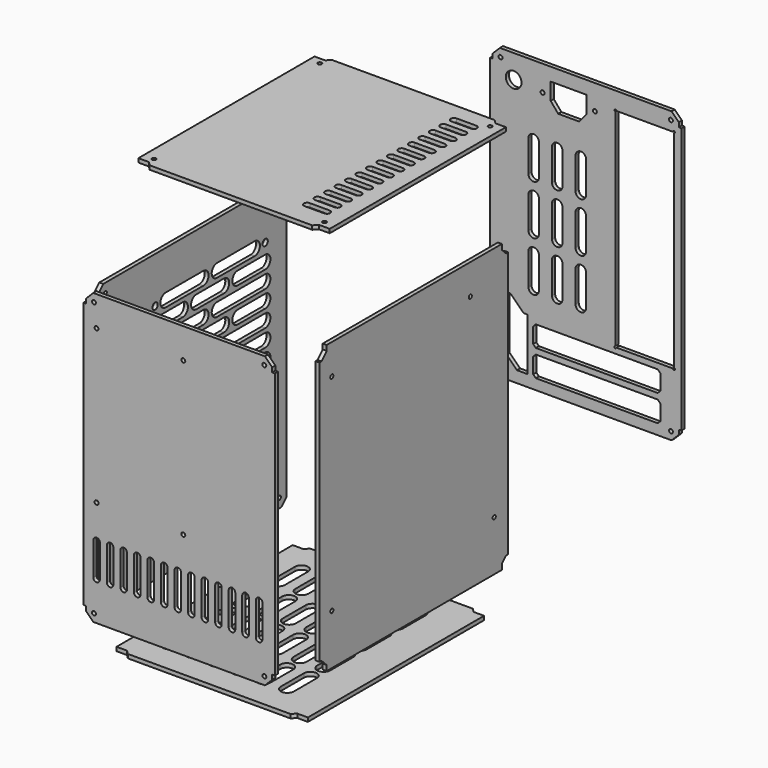
from build123d import *

# Parameters (mm, degrees)
F0_R      = 1.5
F1_DEPTH  = 3
F3_R      = 1.5
F4_DEPTH  = 3
F7_DEPTH  = 3
F9_R      = 1.5
F10_DEPTH = 25
F12_R     = 1.5
F13_DEPTH = 3
F15_R     = 2.5
F16_DEPTH = 25
F18_R     = 1.5
F19_DEPTH = 3
F23_DEPTH = 3
F27_DEPTH = 25
F28_R     = 1.5
F29_DEPTH = 3
F31_W     = 97
F31_H     = 15.9
F32_R     = 1.5
F32_R_2   = 6
F33_DEPTH = 25
F34_SIZE  = 2
F36_DEPTH = 25


# Not quite as in the source:
# - a feature names something its author has since deleted; it is built from what else it names


with BuildPart() as f1:
    # F0 (on Front) → F1 (new body)
    with BuildSketch(Plane.XZ):
        Polygon((-73.4445467208, 95.1760702261), (-75.4445467208, 95.1760702261), (-75.4445467208, -6.3239297739), (70.5554532792, -6.3239297739), (70.5554532792, 95.1760702261), (68.5554532792, 95.1760702261), (68.5554532792, 98.6760702261), (63.0554532792, 104.1760702261), (-67.9445467208, 104.1760702261), (-73.4445467208, 98.6760702261), align=None)
        with Locations((-67.4445467208, 98.1760702261)):
            Circle(F0_R, mode=Mode.SUBTRACT)
        with Locations((62.5554532792, 98.1760702261)):
            Circle(F0_R, mode=Mode.SUBTRACT)
    extrude(amount=F1_DEPTH)

    # F2: F1 across face


with BuildPart() as f1_1:
    add(f1.part)
    add(f1.part.mirror(Plane(origin=(-2.4445467208, -1.5, -6.3239297739), x_dir=(1, 0, 0), z_dir=(0, 0, -1))))

    # F3 (on face) → F4 (cut)
    with BuildSketch(Plane.XZ.offset(3)):
        with Locations((0.7554532792, 81.1760702261)):
            Circle(F3_R)
        with Locations((-65.4445467208, 81.1760702261)):
            Circle(F3_R)
        with Locations((-65.4445467208, -35.8239297739)):
            Circle(F3_R)
        with Locations((0.7554532792, -35.8239297739)):
            Circle(F3_R)
        with BuildLine():
            ThreePointArc((-67.9445467208, -86.8239297739), (-65.4445467208, -89.3239297739), (-62.9445467208, -86.8239297739))
            Line((-62.9445467208, -86.8239297739), (-62.9445467208, -61.8239297739))
            ThreePointArc((-62.9445467208, -61.8239297739), (-65.4445467208, -59.3239297739), (-67.9445467208, -61.8239297739))
            Line((-67.9445467208, -61.8239297739), (-67.9445467208, -86.8239297739))
        make_face()
        with BuildLine():
            ThreePointArc((-57.6115467208, -86.8239297739), (-55.1115467208, -89.3239297739), (-52.6115467208, -86.8239297739))
            Line((-52.6115467208, -86.8239297739), (-52.6115467208, -61.8239297739))
            ThreePointArc((-52.6115467208, -61.8239297739), (-55.1115467208, -59.3239297739), (-57.6115467208, -61.8239297739))
            Line((-57.6115467208, -61.8239297739), (-57.6115467208, -86.8239297739))
        make_face()
        with BuildLine():
            ThreePointArc((-47.2785467208, -86.8239297739), (-44.7785467208, -89.3239297739), (-42.2785467208, -86.8239297739))
            Line((-42.2785467208, -86.8239297739), (-42.2785467208, -61.8239297739))
            ThreePointArc((-42.2785467208, -61.8239297739), (-44.7785467208, -59.3239297739), (-47.2785467208, -61.8239297739))
            Line((-47.2785467208, -61.8239297739), (-47.2785467208, -86.8239297739))
        make_face()
        with BuildLine():
            ThreePointArc((-36.9455467208, -86.8239297739), (-34.4455467208, -89.3239297739), (-31.9455467208, -86.8239297739))
            Line((-31.9455467208, -86.8239297739), (-31.9455467208, -61.8239297739))
            ThreePointArc((-31.9455467208, -61.8239297739), (-34.4455467208, -59.3239297739), (-36.9455467208, -61.8239297739))
            Line((-36.9455467208, -61.8239297739), (-36.9455467208, -86.8239297739))
        make_face()
        with BuildLine():
            ThreePointArc((-26.6125467208, -86.8239297739), (-24.1125467208, -89.3239297739), (-21.6125467208, -86.8239297739))
            Line((-21.6125467208, -86.8239297739), (-21.6125467208, -61.8239297739))
            ThreePointArc((-21.6125467208, -61.8239297739), (-24.1125467208, -59.3239297739), (-26.6125467208, -61.8239297739))
            Line((-26.6125467208, -61.8239297739), (-26.6125467208, -86.8239297739))
        make_face()
        with BuildLine():
            ThreePointArc((-16.2795467208, -86.8239297739), (-13.7795467208, -89.3239297739), (-11.2795467208, -86.8239297739))
            Line((-11.2795467208, -86.8239297739), (-11.2795467208, -61.8239297739))
            ThreePointArc((-11.2795467208, -61.8239297739), (-13.7795467208, -59.3239297739), (-16.2795467208, -61.8239297739))
            Line((-16.2795467208, -61.8239297739), (-16.2795467208, -86.8239297739))
        make_face()
        with BuildLine():
            ThreePointArc((-5.9465467208, -86.8239297739), (-3.4465467208, -89.3239297739), (-0.9465467208, -86.8239297739))
            Line((-0.9465467208, -86.8239297739), (-0.9465467208, -61.8239297739))
            ThreePointArc((-0.9465467208, -61.8239297739), (-3.4465467208, -59.3239297739), (-5.9465467208, -61.8239297739))
            Line((-5.9465467208, -61.8239297739), (-5.9465467208, -86.8239297739))
        make_face()
        with BuildLine():
            ThreePointArc((4.3864532792, -86.8239297739), (6.8864532792, -89.3239297739), (9.3864532792, -86.8239297739))
            Line((9.3864532792, -86.8239297739), (9.3864532792, -61.8239297739))
            ThreePointArc((9.3864532792, -61.8239297739), (6.8864532792, -59.3239297739), (4.3864532792, -61.8239297739))
            Line((4.3864532792, -61.8239297739), (4.3864532792, -86.8239297739))
        make_face()
        with BuildLine():
            ThreePointArc((14.7194532792, -86.8239297739), (17.2194532792, -89.3239297739), (19.7194532792, -86.8239297739))
            Line((19.7194532792, -86.8239297739), (19.7194532792, -61.8239297739))
            ThreePointArc((19.7194532792, -61.8239297739), (17.2194532792, -59.3239297739), (14.7194532792, -61.8239297739))
            Line((14.7194532792, -61.8239297739), (14.7194532792, -86.8239297739))
        make_face()
        with BuildLine():
            ThreePointArc((25.0524532792, -86.8239297739), (27.5524532792, -89.3239297739), (30.0524532792, -86.8239297739))
            Line((30.0524532792, -86.8239297739), (30.0524532792, -61.8239297739))
            ThreePointArc((30.0524532792, -61.8239297739), (27.5524532792, -59.3239297739), (25.0524532792, -61.8239297739))
            Line((25.0524532792, -61.8239297739), (25.0524532792, -86.8239297739))
        make_face()
        with BuildLine():
            ThreePointArc((35.3854532792, -86.8239297739), (37.8854532792, -89.3239297739), (40.3854532792, -86.8239297739))
            Line((40.3854532792, -86.8239297739), (40.3854532792, -61.8239297739))
            ThreePointArc((40.3854532792, -61.8239297739), (37.8854532792, -59.3239297739), (35.3854532792, -61.8239297739))
            Line((35.3854532792, -61.8239297739), (35.3854532792, -86.8239297739))
        make_face()
        with BuildLine():
            ThreePointArc((45.7184532792, -86.8239297739), (48.2184532792, -89.3239297739), (50.7184532792, -86.8239297739))
            Line((50.7184532792, -86.8239297739), (50.7184532792, -61.8239297739))
            ThreePointArc((50.7184532792, -61.8239297739), (48.2184532792, -59.3239297739), (45.7184532792, -61.8239297739))
            Line((45.7184532792, -61.8239297739), (45.7184532792, -86.8239297739))
        make_face()
        with BuildLine():
            ThreePointArc((56.0514532792, -86.8239297739), (58.5514532792, -89.3239297739), (61.0514532792, -86.8239297739))
            Line((61.0514532792, -86.8239297739), (61.0514532792, -61.8239297739))
            ThreePointArc((61.0514532792, -61.8239297739), (58.5514532792, -59.3239297739), (56.0514532792, -61.8239297739))
            Line((56.0514532792, -61.8239297739), (56.0514532792, -86.8239297739))
        make_face()
    extrude(amount=-F4_DEPTH, mode=Mode.SUBTRACT)


with BuildPart() as f7:
    # F6 (on offset) → F7 (new body)
    with BuildSketch(Plane.YZ.offset(80)):
        Polygon((197.9221091728, 104.5042446256), (30.9221091728, 104.5042446256), (30.9221091728, 100.5042446256), (25.9221091728, 95.5042446256), (23.9221091728, 95.5042446256), (23.9221091728, -4.9957553744), (203.9221091728, -4.9957553744), (203.9221091728, 96.5042446256), (201.9221091728, 96.5042446256), (197.9221091728, 100.5042446256), align=None)
    extrude(amount=F7_DEPTH)

    # F8: F7 across face


with BuildPart() as f7_1:
    add(f7.part)
    add(f7.part.mirror(Plane(origin=(81.5, 113.9221091728, -4.9957553744), x_dir=(1, 0, 0), z_dir=(0, 0, -1))))

    # F9 (on face) → F10 (cut)
    with BuildSketch(Plane(origin=(80, 0, 0), x_dir=(0, -1, 0), z_dir=(-1, 0, 0))):
        with Locations((-190.7221091728, -76.0957553744)):
            Circle(F9_R)
        with Locations((-35.8221091728, -76.0957553744)):
            Circle(F9_R)
        with Locations((-167.9221091728, 81.3042446256)):
            Circle(F9_R)
        with Locations((-35.8221091728, 81.3042446256)):
            Circle(F9_R)
    extrude(amount=-F10_DEPTH, mode=Mode.SUBTRACT)


with BuildPart() as f13:
    # F12 (on offset) → F13 (new body)
    with BuildSketch(Plane.YZ.offset(-96)):
        Polygon((212.7864820957, 80.4807467597), (207.7864820957, 85.4807467597), (37.7864820957, 85.4807467597), (32.7864820957, 80.4807467597), (32.7864820957, -24.0192532403), (212.7864820957, -24.0192532403), align=None)
        with Locations((39.7864820957, 78.4807467597)):
            Circle(F12_R, mode=Mode.SUBTRACT)
        with Locations((205.7864820957, 78.4807467597)):
            Circle(F12_R, mode=Mode.SUBTRACT)
    extrude(amount=F13_DEPTH)

    # F14: F13 across face


with BuildPart() as f13_1:
    add(f13.part)
    add(f13.part.mirror(Plane(origin=(-94.5, 122.7864820957, -24.0192532403), x_dir=(1, 0, 0), z_dir=(0, 0, -1))))

    # F15 (on face) → F16 (cut)
    with BuildSketch(Plane(origin=(-96, 0, 0), x_dir=(0, -1, 0), z_dir=(-1, 0, 0))):
        with Locations((-192.2864820957, 50.4807467597)):
            Circle(F15_R)
        with Locations((-87.2864820957, 50.4807467597)):
            Circle(F15_R)
        with BuildLine():
            ThreePointArc((-182.2864820957, 55.4807467597), (-187.2864820957, 50.4807467597), (-182.2864820957, 45.4807467597))
            Line((-182.2864820957, 45.4807467597), (-146.2864820957, 45.4807467597))
            ThreePointArc((-146.2864820957, 45.4807467597), (-141.2864820957, 50.4807467597), (-146.2864820957, 55.4807467597))
            Line((-146.2864820957, 55.4807467597), (-182.2864820957, 55.4807467597))
        make_face()
        with BuildLine():
            ThreePointArc((-133.2864820957, 55.4807467597), (-138.2864820957, 50.4807467597), (-133.2864820957, 45.4807467597))
            Line((-133.2864820957, 45.4807467597), (-97.2864820957, 45.4807467597))
            ThreePointArc((-97.2864820957, 45.4807467597), (-92.2864820957, 50.4807467597), (-97.2864820957, 55.4807467597))
            Line((-97.2864820957, 55.4807467597), (-133.2864820957, 55.4807467597))
        make_face()
        with BuildLine():
            ThreePointArc((-192.2864820957, 42.3557467597), (-197.2864820957, 37.3557467597), (-192.2864820957, 32.3557467597))
            Line((-192.2864820957, 32.3557467597), (-165.9531487624, 32.3557467597))
            ThreePointArc((-165.9531487624, 32.3557467597), (-160.9531487624, 37.3557467597), (-165.9531487624, 42.3557467597))
            Line((-165.9531487624, 42.3557467597), (-192.2864820957, 42.3557467597))
        make_face()
        with BuildLine():
            ThreePointArc((-152.9531487624, 42.3557467597), (-157.9531487624, 37.3557467597), (-152.9531487624, 32.3557467597))
            Line((-152.9531487624, 32.3557467597), (-126.6198154291, 32.3557467597))
            ThreePointArc((-126.6198154291, 32.3557467597), (-121.6198154291, 37.3557467597), (-126.6198154291, 42.3557467597))
            Line((-126.6198154291, 42.3557467597), (-152.9531487624, 42.3557467597))
        make_face()
        with BuildLine():
            ThreePointArc((-113.6198154291, 42.3557467597), (-118.6198154291, 37.3557467597), (-113.6198154291, 32.3557467597))
            Line((-113.6198154291, 32.3557467597), (-87.2864820957, 32.3557467597))
            ThreePointArc((-87.2864820957, 32.3557467597), (-82.2864820957, 37.3557467597), (-87.2864820957, 42.3557467597))
            Line((-87.2864820957, 42.3557467597), (-113.6198154291, 42.3557467597))
        make_face()
        with BuildLine():
            ThreePointArc((-192.2864820957, 29.2307467597), (-197.2864820957, 24.2307467597), (-192.2864820957, 19.2307467597))
            Line((-192.2864820957, 19.2307467597), (-146.2864820957, 19.2307467597))
            ThreePointArc((-146.2864820957, 19.2307467597), (-141.2864820957, 24.2307467597), (-146.2864820957, 29.2307467597))
            Line((-146.2864820957, 29.2307467597), (-192.2864820957, 29.2307467597))
        make_face()
        with BuildLine():
            ThreePointArc((-133.2864820957, 29.2307467597), (-138.2864820957, 24.2307467597), (-133.2864820957, 19.2307467597))
            Line((-133.2864820957, 19.2307467597), (-87.2864820957, 19.2307467597))
            ThreePointArc((-87.2864820957, 19.2307467597), (-82.2864820957, 24.2307467597), (-87.2864820957, 29.2307467597))
            Line((-87.2864820957, 29.2307467597), (-133.2864820957, 29.2307467597))
        make_face()
        with BuildLine():
            ThreePointArc((-192.2864820957, 16.1057467597), (-197.2864820957, 11.1057467597), (-192.2864820957, 6.1057467597))
            Line((-192.2864820957, 6.1057467597), (-165.9531487624, 6.1057467597))
            ThreePointArc((-165.9531487624, 6.1057467597), (-160.9531487624, 11.1057467597), (-165.9531487624, 16.1057467597))
            Line((-165.9531487624, 16.1057467597), (-192.2864820957, 16.1057467597))
        make_face()
        with BuildLine():
            ThreePointArc((-152.9531487624, 16.1057467597), (-157.9531487624, 11.1057467597), (-152.9531487624, 6.1057467597))
            Line((-152.9531487624, 6.1057467597), (-126.6198154291, 6.1057467597))
            ThreePointArc((-126.6198154291, 6.1057467597), (-121.6198154291, 11.1057467597), (-126.6198154291, 16.1057467597))
            Line((-126.6198154291, 16.1057467597), (-152.9531487624, 16.1057467597))
        make_face()
        with BuildLine():
            ThreePointArc((-113.6198154291, 16.1057467597), (-118.6198154291, 11.1057467597), (-113.6198154291, 6.1057467597))
            Line((-113.6198154291, 6.1057467597), (-87.2864820957, 6.1057467597))
            ThreePointArc((-87.2864820957, 6.1057467597), (-82.2864820957, 11.1057467597), (-87.2864820957, 16.1057467597))
            Line((-87.2864820957, 16.1057467597), (-113.6198154291, 16.1057467597))
        make_face()
        with BuildLine():
            ThreePointArc((-192.2864820957, 2.9807467597), (-197.2864820957, -2.0192532403), (-192.2864820957, -7.0192532403))
            Line((-192.2864820957, -7.0192532403), (-146.2864820957, -7.0192532403))
            ThreePointArc((-146.2864820957, -7.0192532403), (-141.2864820957, -2.0192532403), (-146.2864820957, 2.9807467597))
            Line((-146.2864820957, 2.9807467597), (-192.2864820957, 2.9807467597))
        make_face()
        with BuildLine():
            ThreePointArc((-133.2864820957, 2.9807467597), (-138.2864820957, -2.0192532403), (-133.2864820957, -7.0192532403))
            Line((-133.2864820957, -7.0192532403), (-87.2864820957, -7.0192532403))
            ThreePointArc((-87.2864820957, -7.0192532403), (-82.2864820957, -2.0192532403), (-87.2864820957, 2.9807467597))
            Line((-87.2864820957, 2.9807467597), (-133.2864820957, 2.9807467597))
        make_face()
        with BuildLine():
            ThreePointArc((-192.2864820957, -10.1442532403), (-197.2864820957, -15.1442532403), (-192.2864820957, -20.1442532403))
            Line((-192.2864820957, -20.1442532403), (-165.9531487624, -20.1442532403))
            ThreePointArc((-165.9531487624, -20.1442532403), (-160.9531487624, -15.1442532403), (-165.9531487624, -10.1442532403))
            Line((-165.9531487624, -10.1442532403), (-192.2864820957, -10.1442532403))
        make_face()
        with BuildLine():
            ThreePointArc((-152.9531487624, -10.1442532403), (-157.9531487624, -15.1442532403), (-152.9531487624, -20.1442532403))
            Line((-152.9531487624, -20.1442532403), (-126.6198154291, -20.1442532403))
            ThreePointArc((-126.6198154291, -20.1442532403), (-121.6198154291, -15.1442532403), (-126.6198154291, -10.1442532403))
            Line((-126.6198154291, -10.1442532403), (-152.9531487624, -10.1442532403))
        make_face()
        with BuildLine():
            ThreePointArc((-113.6198154291, -10.1442532403), (-118.6198154291, -15.1442532403), (-113.6198154291, -20.1442532403))
            Line((-113.6198154291, -20.1442532403), (-87.2864820957, -20.1442532403))
            ThreePointArc((-87.2864820957, -20.1442532403), (-82.2864820957, -15.1442532403), (-87.2864820957, -10.1442532403))
            Line((-87.2864820957, -10.1442532403), (-113.6198154291, -10.1442532403))
        make_face()
        with BuildLine():
            ThreePointArc((-192.2864820957, -23.2692532403), (-197.2864820957, -28.2692532403), (-192.2864820957, -33.2692532403))
            Line((-192.2864820957, -33.2692532403), (-146.2864820957, -33.2692532403))
            ThreePointArc((-146.2864820957, -33.2692532403), (-141.2864820957, -28.2692532403), (-146.2864820957, -23.2692532403))
            Line((-146.2864820957, -23.2692532403), (-192.2864820957, -23.2692532403))
        make_face()
        with BuildLine():
            ThreePointArc((-133.2864820957, -23.2692532403), (-138.2864820957, -28.2692532403), (-133.2864820957, -33.2692532403))
            Line((-133.2864820957, -33.2692532403), (-87.2864820957, -33.2692532403))
            ThreePointArc((-87.2864820957, -33.2692532403), (-82.2864820957, -28.2692532403), (-87.2864820957, -23.2692532403))
            Line((-87.2864820957, -23.2692532403), (-133.2864820957, -23.2692532403))
        make_face()
        with BuildLine():
            ThreePointArc((-192.2864820957, -36.3942532403), (-197.2864820957, -41.3942532403), (-192.2864820957, -46.3942532403))
            Line((-192.2864820957, -46.3942532403), (-165.9531487624, -46.3942532403))
            ThreePointArc((-165.9531487624, -46.3942532403), (-160.9531487624, -41.3942532403), (-165.9531487624, -36.3942532403))
            Line((-165.9531487624, -36.3942532403), (-192.2864820957, -36.3942532403))
        make_face()
        with BuildLine():
            ThreePointArc((-152.9531487624, -36.3942532403), (-157.9531487624, -41.3942532403), (-152.9531487624, -46.3942532403))
            Line((-152.9531487624, -46.3942532403), (-126.6198154291, -46.3942532403))
            ThreePointArc((-126.6198154291, -46.3942532403), (-121.6198154291, -41.3942532403), (-126.6198154291, -36.3942532403))
            Line((-126.6198154291, -36.3942532403), (-152.9531487624, -36.3942532403))
        make_face()
        with BuildLine():
            ThreePointArc((-113.6198154291, -36.3942532403), (-118.6198154291, -41.3942532403), (-113.6198154291, -46.3942532403))
            Line((-113.6198154291, -46.3942532403), (-87.2864820957, -46.3942532403))
            ThreePointArc((-87.2864820957, -46.3942532403), (-82.2864820957, -41.3942532403), (-87.2864820957, -36.3942532403))
            Line((-87.2864820957, -36.3942532403), (-113.6198154291, -36.3942532403))
        make_face()
        with BuildLine():
            ThreePointArc((-182.2864820957, -49.5192532403), (-187.2864820957, -54.5192532403), (-182.2864820957, -59.5192532403))
            Line((-182.2864820957, -59.5192532403), (-146.2864820957, -59.5192532403))
            ThreePointArc((-146.2864820957, -59.5192532403), (-141.2864820957, -54.5192532403), (-146.2864820957, -49.5192532403))
            Line((-146.2864820957, -49.5192532403), (-182.2864820957, -49.5192532403))
        make_face()
        with BuildLine():
            ThreePointArc((-133.2864820957, -49.5192532403), (-138.2864820957, -54.5192532403), (-133.2864820957, -59.5192532403))
            Line((-133.2864820957, -59.5192532403), (-97.2864820957, -59.5192532403))
            ThreePointArc((-97.2864820957, -59.5192532403), (-92.2864820957, -54.5192532403), (-97.2864820957, -49.5192532403))
            Line((-97.2864820957, -49.5192532403), (-133.2864820957, -49.5192532403))
        make_face()
        with Locations((-192.2864820957, -54.5192532403)):
            Circle(F15_R)
        with Locations((-87.2864820957, -54.5192532403)):
            Circle(F15_R)
    extrude(amount=-F16_DEPTH, mode=Mode.SUBTRACT)


with BuildPart() as f19:
    # F18 (on offset) → F19 (new body)
    with BuildSketch(Plane.XY.offset(155)):
        Polygon((54.9777505851, 152.8661787467), (-91.0222494149, 152.8661787467), (-91.0222494149, 68.8661787467), (-83.0222494149, 68.8661787467), (-80.0222494149, 65.8661787467), (43.9777505851, 65.8661787467), (46.9777505851, 68.8661787467), (54.9777505851, 68.8661787467), align=None)
        with Locations((-83.0222494149, 73.8661787467)):
            Circle(F18_R, mode=Mode.SUBTRACT)
        with Locations((46.9777505851, 73.8661787467)):
            Circle(F18_R, mode=Mode.SUBTRACT)
    extrude(amount=F19_DEPTH)

    # F20: F19 across face


with BuildPart() as f19_1:
    add(f19.part)
    add(f19.part.mirror(Plane(origin=(-18.0222494149, 152.8661787467, 156.5), x_dir=(-1, 0, 0), z_dir=(0, 1, 0))))

    # F35 (on face) → F36 (cut)
    with BuildSketch(Plane.XY.offset(158)):
        with BuildLine():
            ThreePointArc((24.9777505851, 227.3661787467), (22.4777505851, 224.8661787467), (24.9777505851, 222.3661787467))
            Line((24.9777505851, 222.3661787467), (39.9777505851, 222.3661787467))
            ThreePointArc((39.9777505851, 222.3661787467), (42.4777505851, 224.8661787467), (39.9777505851, 227.3661787467))
            Line((39.9777505851, 227.3661787467), (24.9777505851, 227.3661787467))
        make_face()
        with BuildLine():
            ThreePointArc((24.9777505851, 217.3661787467), (22.4777505851, 214.8661787467), (24.9777505851, 212.3661787467))
            Line((24.9777505851, 212.3661787467), (39.9777505851, 212.3661787467))
            ThreePointArc((39.9777505851, 212.3661787467), (42.4777505851, 214.8661787467), (39.9777505851, 217.3661787467))
            Line((39.9777505851, 217.3661787467), (24.9777505851, 217.3661787467))
        make_face()
        with BuildLine():
            ThreePointArc((24.9777505851, 207.3661787467), (22.4777505851, 204.8661787467), (24.9777505851, 202.3661787467))
            Line((24.9777505851, 202.3661787467), (39.9777505851, 202.3661787467))
            ThreePointArc((39.9777505851, 202.3661787467), (42.4777505851, 204.8661787467), (39.9777505851, 207.3661787467))
            Line((39.9777505851, 207.3661787467), (24.9777505851, 207.3661787467))
        make_face()
        with BuildLine():
            ThreePointArc((24.9777505851, 197.3661787467), (22.4777505851, 194.8661787467), (24.9777505851, 192.3661787467))
            Line((24.9777505851, 192.3661787467), (39.9777505851, 192.3661787467))
            ThreePointArc((39.9777505851, 192.3661787467), (42.4777505851, 194.8661787467), (39.9777505851, 197.3661787467))
            Line((39.9777505851, 197.3661787467), (24.9777505851, 197.3661787467))
        make_face()
        with BuildLine():
            ThreePointArc((24.9777505851, 187.3661787467), (22.4777505851, 184.8661787467), (24.9777505851, 182.3661787467))
            Line((24.9777505851, 182.3661787467), (39.9777505851, 182.3661787467))
            ThreePointArc((39.9777505851, 182.3661787467), (42.4777505851, 184.8661787467), (39.9777505851, 187.3661787467))
            Line((39.9777505851, 187.3661787467), (24.9777505851, 187.3661787467))
        make_face()
        with BuildLine():
            ThreePointArc((24.9777505851, 177.3661787467), (22.4777505851, 174.8661787467), (24.9777505851, 172.3661787467))
            Line((24.9777505851, 172.3661787467), (39.9777505851, 172.3661787467))
            ThreePointArc((39.9777505851, 172.3661787467), (42.4777505851, 174.8661787467), (39.9777505851, 177.3661787467))
            Line((39.9777505851, 177.3661787467), (24.9777505851, 177.3661787467))
        make_face()
        with BuildLine():
            ThreePointArc((24.9777505851, 167.3661787467), (22.4777505851, 164.8661787467), (24.9777505851, 162.3661787467))
            Line((24.9777505851, 162.3661787467), (39.9777505851, 162.3661787467))
            ThreePointArc((39.9777505851, 162.3661787467), (42.4777505851, 164.8661787467), (39.9777505851, 167.3661787467))
            Line((39.9777505851, 167.3661787467), (24.9777505851, 167.3661787467))
        make_face()
        with BuildLine():
            ThreePointArc((24.9777505851, 157.3661787467), (22.4777505851, 154.8661787467), (24.9777505851, 152.3661787467))
            Line((24.9777505851, 152.3661787467), (39.9777505851, 152.3661787467))
            ThreePointArc((39.9777505851, 152.3661787467), (42.4777505851, 154.8661787467), (39.9777505851, 157.3661787467))
            Line((39.9777505851, 157.3661787467), (24.9777505851, 157.3661787467))
        make_face()
        with BuildLine():
            ThreePointArc((24.9777505851, 147.3661787467), (22.4777505851, 144.8661787467), (24.9777505851, 142.3661787467))
            Line((24.9777505851, 142.3661787467), (39.9777505851, 142.3661787467))
            ThreePointArc((39.9777505851, 142.3661787467), (42.4777505851, 144.8661787467), (39.9777505851, 147.3661787467))
            Line((39.9777505851, 147.3661787467), (24.9777505851, 147.3661787467))
        make_face()
        with BuildLine():
            ThreePointArc((24.9777505851, 137.3661787467), (22.4777505851, 134.8661787467), (24.9777505851, 132.3661787467))
            Line((24.9777505851, 132.3661787467), (39.9777505851, 132.3661787467))
            ThreePointArc((39.9777505851, 132.3661787467), (42.4777505851, 134.8661787467), (39.9777505851, 137.3661787467))
            Line((39.9777505851, 137.3661787467), (24.9777505851, 137.3661787467))
        make_face()
        with BuildLine():
            ThreePointArc((24.9777505851, 127.3661787467), (22.4777505851, 124.8661787467), (24.9777505851, 122.3661787467))
            Line((24.9777505851, 122.3661787467), (39.9777505851, 122.3661787467))
            ThreePointArc((39.9777505851, 122.3661787467), (42.4777505851, 124.8661787467), (39.9777505851, 127.3661787467))
            Line((39.9777505851, 127.3661787467), (24.9777505851, 127.3661787467))
        make_face()
        with BuildLine():
            ThreePointArc((24.9777505851, 117.3661787467), (22.4777505851, 114.8661787467), (24.9777505851, 112.3661787467))
            Line((24.9777505851, 112.3661787467), (39.9777505851, 112.3661787467))
            ThreePointArc((39.9777505851, 112.3661787467), (42.4777505851, 114.8661787467), (39.9777505851, 117.3661787467))
            Line((39.9777505851, 117.3661787467), (24.9777505851, 117.3661787467))
        make_face()
        with BuildLine():
            ThreePointArc((24.9777505851, 107.3661787467), (22.4777505851, 104.8661787467), (24.9777505851, 102.3661787467))
            Line((24.9777505851, 102.3661787467), (39.9777505851, 102.3661787467))
            ThreePointArc((39.9777505851, 102.3661787467), (42.4777505851, 104.8661787467), (39.9777505851, 107.3661787467))
            Line((39.9777505851, 107.3661787467), (24.9777505851, 107.3661787467))
        make_face()
        with BuildLine():
            ThreePointArc((24.9777505851, 97.3661787467), (22.4777505851, 94.8661787467), (24.9777505851, 92.3661787467))
            Line((24.9777505851, 92.3661787467), (39.9777505851, 92.3661787467))
            ThreePointArc((39.9777505851, 92.3661787467), (42.4777505851, 94.8661787467), (39.9777505851, 97.3661787467))
            Line((39.9777505851, 97.3661787467), (24.9777505851, 97.3661787467))
        make_face()
        with BuildLine():
            ThreePointArc((24.9777505851, 87.3661787467), (22.4777505851, 84.8661787467), (24.9777505851, 82.3661787467))
            Line((24.9777505851, 82.3661787467), (39.9777505851, 82.3661787467))
            ThreePointArc((39.9777505851, 82.3661787467), (42.4777505851, 84.8661787467), (39.9777505851, 87.3661787467))
            Line((39.9777505851, 87.3661787467), (24.9777505851, 87.3661787467))
        make_face()
    extrude(amount=-F36_DEPTH, mode=Mode.SUBTRACT)


with BuildPart() as f23:
    # F22 (on offset) → F23 (new body)
    with BuildSketch(Plane.XY.offset(-153)):
        Polygon((-68.9245462418, 30.4242391139), (-65.9245462418, 27.4242391139), (58.0754537582, 27.4242391139), (61.0754537582, 30.4242391139), (69.0754537582, 30.4242391139), (69.0754537582, 114.4242391139), (-76.9245462418, 114.4242391139), (-76.9245462418, 30.4242391139), align=None)
    extrude(amount=F23_DEPTH)

    # F24: F23 across face


with BuildPart() as f23_1:
    add(f23.part)
    add(f23.part.mirror(Plane(origin=(-3.9245462418, 114.4242391139, -151.5), x_dir=(-1, 0, 0), z_dir=(0, 1, 0))))

    # F26 (on face) → F27 (cut)
    with BuildSketch(Plane(origin=(0, 0, -153), x_dir=(1, 0, 0), z_dir=(0, 0, -1))):
        with BuildLine():
            ThreePointArc((-58.4245462418, -177.4242391139), (-53.4245462418, -182.4242391139), (-48.4245462418, -177.4242391139))
            Line((-48.4245462418, -177.4242391139), (-48.4245462418, -155.4242391139))
            ThreePointArc((-48.4245462418, -155.4242391139), (-53.4245462418, -150.4242391139), (-58.4245462418, -155.4242391139))
            Line((-58.4245462418, -155.4242391139), (-58.4245462418, -177.4242391139))
        make_face()
        with BuildLine():
            ThreePointArc((-58.4245462418, -142.7575724473), (-53.4245462418, -147.7575724473), (-48.4245462418, -142.7575724473))
            Line((-48.4245462418, -142.7575724473), (-48.4245462418, -120.7575724473))
            ThreePointArc((-48.4245462418, -120.7575724473), (-53.4245462418, -115.7575724473), (-58.4245462418, -120.7575724473))
            Line((-58.4245462418, -120.7575724473), (-58.4245462418, -142.7575724473))
        make_face()
        with BuildLine():
            ThreePointArc((-58.4245462418, -108.0909057806), (-53.4245462418, -113.0909057806), (-48.4245462418, -108.0909057806))
            Line((-48.4245462418, -108.0909057806), (-48.4245462418, -86.0909057806))
            ThreePointArc((-48.4245462418, -86.0909057806), (-53.4245462418, -81.0909057806), (-58.4245462418, -86.0909057806))
            Line((-58.4245462418, -86.0909057806), (-58.4245462418, -108.0909057806))
        make_face()
        with BuildLine():
            ThreePointArc((-58.4245462418, -73.4242391139), (-53.4245462418, -78.4242391139), (-48.4245462418, -73.4242391139))
            Line((-48.4245462418, -73.4242391139), (-48.4245462418, -51.4242391139))
            ThreePointArc((-48.4245462418, -51.4242391139), (-53.4245462418, -46.4242391139), (-58.4245462418, -51.4242391139))
            Line((-58.4245462418, -51.4242391139), (-58.4245462418, -73.4242391139))
        make_face()
        with BuildLine():
            ThreePointArc((-40.4245462418, -177.4242391139), (-35.4245462418, -182.4242391139), (-30.4245462418, -177.4242391139))
            Line((-30.4245462418, -177.4242391139), (-30.4245462418, -155.4242391139))
            ThreePointArc((-30.4245462418, -155.4242391139), (-35.4245462418, -150.4242391139), (-40.4245462418, -155.4242391139))
            Line((-40.4245462418, -155.4242391139), (-40.4245462418, -177.4242391139))
        make_face()
        with BuildLine():
            ThreePointArc((-40.4245462418, -142.7575724473), (-35.4245462418, -147.7575724473), (-30.4245462418, -142.7575724473))
            Line((-30.4245462418, -142.7575724473), (-30.4245462418, -120.7575724473))
            ThreePointArc((-30.4245462418, -120.7575724473), (-35.4245462418, -115.7575724473), (-40.4245462418, -120.7575724473))
            Line((-40.4245462418, -120.7575724473), (-40.4245462418, -142.7575724473))
        make_face()
        with BuildLine():
            ThreePointArc((-40.4245462418, -108.0909057806), (-35.4245462418, -113.0909057806), (-30.4245462418, -108.0909057806))
            Line((-30.4245462418, -108.0909057806), (-30.4245462418, -86.0909057806))
            ThreePointArc((-30.4245462418, -86.0909057806), (-35.4245462418, -81.0909057806), (-40.4245462418, -86.0909057806))
            Line((-40.4245462418, -86.0909057806), (-40.4245462418, -108.0909057806))
        make_face()
        with BuildLine():
            ThreePointArc((-40.4245462418, -73.4242391139), (-35.4245462418, -78.4242391139), (-30.4245462418, -73.4242391139))
            Line((-30.4245462418, -73.4242391139), (-30.4245462418, -51.4242391139))
            ThreePointArc((-30.4245462418, -51.4242391139), (-35.4245462418, -46.4242391139), (-40.4245462418, -51.4242391139))
            Line((-40.4245462418, -51.4242391139), (-40.4245462418, -73.4242391139))
        make_face()
        with BuildLine():
            ThreePointArc((-22.4245462418, -177.4242391139), (-17.4245462418, -182.4242391139), (-12.4245462418, -177.4242391139))
            Line((-12.4245462418, -177.4242391139), (-12.4245462418, -155.4242391139))
            ThreePointArc((-12.4245462418, -155.4242391139), (-17.4245462418, -150.4242391139), (-22.4245462418, -155.4242391139))
            Line((-22.4245462418, -155.4242391139), (-22.4245462418, -177.4242391139))
        make_face()
        with BuildLine():
            ThreePointArc((-22.4245462418, -142.7575724473), (-17.4245462418, -147.7575724473), (-12.4245462418, -142.7575724473))
            Line((-12.4245462418, -142.7575724473), (-12.4245462418, -120.7575724473))
            ThreePointArc((-12.4245462418, -120.7575724473), (-17.4245462418, -115.7575724473), (-22.4245462418, -120.7575724473))
            Line((-22.4245462418, -120.7575724473), (-22.4245462418, -142.7575724473))
        make_face()
        with BuildLine():
            ThreePointArc((-22.4245462418, -108.0909057806), (-17.4245462418, -113.0909057806), (-12.4245462418, -108.0909057806))
            Line((-12.4245462418, -108.0909057806), (-12.4245462418, -86.0909057806))
            ThreePointArc((-12.4245462418, -86.0909057806), (-17.4245462418, -81.0909057806), (-22.4245462418, -86.0909057806))
            Line((-22.4245462418, -86.0909057806), (-22.4245462418, -108.0909057806))
        make_face()
        with BuildLine():
            ThreePointArc((-22.4245462418, -73.4242391139), (-17.4245462418, -78.4242391139), (-12.4245462418, -73.4242391139))
            Line((-12.4245462418, -73.4242391139), (-12.4245462418, -51.4242391139))
            ThreePointArc((-12.4245462418, -51.4242391139), (-17.4245462418, -46.4242391139), (-22.4245462418, -51.4242391139))
            Line((-22.4245462418, -51.4242391139), (-22.4245462418, -73.4242391139))
        make_face()
        with BuildLine():
            ThreePointArc((-4.4245462418, -177.4242391139), (0.5754537582, -182.4242391139), (5.5754537582, -177.4242391139))
            Line((5.5754537582, -177.4242391139), (5.5754537582, -155.4242391139))
            ThreePointArc((5.5754537582, -155.4242391139), (0.5754537582, -150.4242391139), (-4.4245462418, -155.4242391139))
            Line((-4.4245462418, -155.4242391139), (-4.4245462418, -177.4242391139))
        make_face()
        with BuildLine():
            ThreePointArc((-4.4245462418, -142.7575724473), (0.5754537582, -147.7575724473), (5.5754537582, -142.7575724473))
            Line((5.5754537582, -142.7575724473), (5.5754537582, -120.7575724473))
            ThreePointArc((5.5754537582, -120.7575724473), (0.5754537582, -115.7575724473), (-4.4245462418, -120.7575724473))
            Line((-4.4245462418, -120.7575724473), (-4.4245462418, -142.7575724473))
        make_face()
        with BuildLine():
            ThreePointArc((-4.4245462418, -108.0909057806), (0.5754537582, -113.0909057806), (5.5754537582, -108.0909057806))
            Line((5.5754537582, -108.0909057806), (5.5754537582, -86.0909057806))
            ThreePointArc((5.5754537582, -86.0909057806), (0.5754537582, -81.0909057806), (-4.4245462418, -86.0909057806))
            Line((-4.4245462418, -86.0909057806), (-4.4245462418, -108.0909057806))
        make_face()
        with BuildLine():
            ThreePointArc((-4.4245462418, -73.4242391139), (0.5754537582, -78.4242391139), (5.5754537582, -73.4242391139))
            Line((5.5754537582, -73.4242391139), (5.5754537582, -51.4242391139))
            ThreePointArc((5.5754537582, -51.4242391139), (0.5754537582, -46.4242391139), (-4.4245462418, -51.4242391139))
            Line((-4.4245462418, -51.4242391139), (-4.4245462418, -73.4242391139))
        make_face()
        with BuildLine():
            ThreePointArc((13.5754537582, -177.4242391139), (18.5754537582, -182.4242391139), (23.5754537582, -177.4242391139))
            Line((23.5754537582, -177.4242391139), (23.5754537582, -155.4242391139))
            ThreePointArc((23.5754537582, -155.4242391139), (18.5754537582, -150.4242391139), (13.5754537582, -155.4242391139))
            Line((13.5754537582, -155.4242391139), (13.5754537582, -177.4242391139))
        make_face()
        with BuildLine():
            ThreePointArc((13.5754537582, -142.7575724473), (18.5754537582, -147.7575724473), (23.5754537582, -142.7575724473))
            Line((23.5754537582, -142.7575724473), (23.5754537582, -120.7575724473))
            ThreePointArc((23.5754537582, -120.7575724473), (18.5754537582, -115.7575724473), (13.5754537582, -120.7575724473))
            Line((13.5754537582, -120.7575724473), (13.5754537582, -142.7575724473))
        make_face()
        with BuildLine():
            ThreePointArc((13.5754537582, -108.0909057806), (18.5754537582, -113.0909057806), (23.5754537582, -108.0909057806))
            Line((23.5754537582, -108.0909057806), (23.5754537582, -86.0909057806))
            ThreePointArc((23.5754537582, -86.0909057806), (18.5754537582, -81.0909057806), (13.5754537582, -86.0909057806))
            Line((13.5754537582, -86.0909057806), (13.5754537582, -108.0909057806))
        make_face()
        with BuildLine():
            ThreePointArc((13.5754537582, -73.4242391139), (18.5754537582, -78.4242391139), (23.5754537582, -73.4242391139))
            Line((23.5754537582, -73.4242391139), (23.5754537582, -51.4242391139))
            ThreePointArc((23.5754537582, -51.4242391139), (18.5754537582, -46.4242391139), (13.5754537582, -51.4242391139))
            Line((13.5754537582, -51.4242391139), (13.5754537582, -73.4242391139))
        make_face()
        with BuildLine():
            ThreePointArc((31.5754537582, -177.4242391139), (36.5754537582, -182.4242391139), (41.5754537582, -177.4242391139))
            Line((41.5754537582, -177.4242391139), (41.5754537582, -155.4242391139))
            ThreePointArc((41.5754537582, -155.4242391139), (36.5754537582, -150.4242391139), (31.5754537582, -155.4242391139))
            Line((31.5754537582, -155.4242391139), (31.5754537582, -177.4242391139))
        make_face()
        with BuildLine():
            ThreePointArc((31.5754537582, -142.7575724473), (36.5754537582, -147.7575724473), (41.5754537582, -142.7575724473))
            Line((41.5754537582, -142.7575724473), (41.5754537582, -120.7575724473))
            ThreePointArc((41.5754537582, -120.7575724473), (36.5754537582, -115.7575724473), (31.5754537582, -120.7575724473))
            Line((31.5754537582, -120.7575724473), (31.5754537582, -142.7575724473))
        make_face()
        with BuildLine():
            ThreePointArc((31.5754537582, -108.0909057806), (36.5754537582, -113.0909057806), (41.5754537582, -108.0909057806))
            Line((41.5754537582, -108.0909057806), (41.5754537582, -86.0909057806))
            ThreePointArc((41.5754537582, -86.0909057806), (36.5754537582, -81.0909057806), (31.5754537582, -86.0909057806))
            Line((31.5754537582, -86.0909057806), (31.5754537582, -108.0909057806))
        make_face()
        with BuildLine():
            ThreePointArc((31.5754537582, -73.4242391139), (36.5754537582, -78.4242391139), (41.5754537582, -73.4242391139))
            Line((41.5754537582, -73.4242391139), (41.5754537582, -51.4242391139))
            ThreePointArc((41.5754537582, -51.4242391139), (36.5754537582, -46.4242391139), (31.5754537582, -51.4242391139))
            Line((31.5754537582, -51.4242391139), (31.5754537582, -73.4242391139))
        make_face()
    extrude(amount=-F27_DEPTH, mode=Mode.SUBTRACT)


with BuildPart() as f29:
    # F28 (on offset) → F29 (new body)
    with BuildSketch(Plane.XZ.offset(-376)):
        Polygon((-64, 109.9973174244), (-66, 109.9973174244), (-66, 8.4973174244), (80, 8.4973174244), (80, 109.9973174244), (78, 109.9973174244), (78, 113.4973174244), (72.5, 118.9973174244), (-58.5, 118.9973174244), (-64, 113.4973174244), align=None)
        with Locations((-58, 112.9973174244)):
            Circle(F28_R, mode=Mode.SUBTRACT)
        with Locations((72, 112.9973174244)):
            Circle(F28_R, mode=Mode.SUBTRACT)
    extrude(amount=F29_DEPTH)

    # F30: F29 across face


with BuildPart() as f29_1:
    add(f29.part)
    add(f29.part.mirror(Plane(origin=(7, 374.5, 8.4973174244), x_dir=(1, 0, 0), z_dir=(0, 0, -1))))

    # F31 (on face) + F32 (on face) → F33 (cut)
    with BuildSketch(Plane(origin=(0, 376, 0), x_dir=(-1, 0, 0), z_dir=(0, 1, 0))):
        with Locations((-15.4, -65.7026825756)):
            Rectangle(F31_W, F31_H)
        with Locations((-15.4, -86.0026825756)):
            Rectangle(F31_W, F31_H)
        Polygon((-29.6, 104.8473174244), (-29.6, 105.5973174244), (-30.35, 105.5973174244), (-73.55, 105.5973174244), (-74.3, 105.5973174244), (-74.3, 104.8473174244), (-74.3, -52.6526825756), (-74.3, -53.4026825756), (-73.55, -53.4026825756), (-30.35, -53.4026825756), (-29.6, -53.4026825756), (-29.6, -52.6526825756), align=None)
        with BuildLine():
            Line((-30.35, 105.5973174244), (-29.6, 105.5973174244))
            Line((-29.6, 105.5973174244), (-29.6, 104.8473174244))
            ThreePointArc((-29.6, 104.8473174244), (-29.0696699141, 106.1276475103), (-30.35, 105.5973174244))
        make_face()
        with BuildLine():
            Line((-74.3, 105.5973174244), (-73.55, 105.5973174244))
            ThreePointArc((-73.55, 105.5973174244), (-74.8303300859, 106.1276475103), (-74.3, 104.8473174244))
            Line((-74.3, 104.8473174244), (-74.3, 105.5973174244))
        make_face()
        with BuildLine():
            ThreePointArc((-30.35, -53.4026825756), (-29.0696699141, -53.9330126615), (-29.6, -52.6526825756))
            Line((-29.6, -52.6526825756), (-29.6, -53.4026825756))
            Line((-29.6, -53.4026825756), (-30.35, -53.4026825756))
        make_face()
        with BuildLine():
            Line((-74.3, -53.4026825756), (-74.3, -52.6526825756))
            ThreePointArc((-74.3, -52.6526825756), (-74.8303300859, -53.9330126615), (-73.55, -53.4026825756))
            Line((-73.55, -53.4026825756), (-74.3, -53.4026825756))
        make_face()
        Polygon((40.5, -53.2526825756), (37.5, -53.2526825756), (37.5, -93.2526825756), (45.5, -93.2526825756), (53.5, -85.2526825756), (53.5, -43.2526825756), (50.5, -43.2526825756), align=None)
    with BuildSketch(Plane(origin=(0, 376, 0), x_dir=(-1, 0, 0), z_dir=(0, 1, 0))):
        with BuildLine():
            ThreePointArc((0.7453302816, 65.4973174244), (-3.2546697184, 69.4973174244), (-7.2546697184, 65.4973174244))
            Line((-7.2546697184, 65.4973174244), (-7.2546697184, 41.4973174244))
            ThreePointArc((-7.2546697184, 41.4973174244), (-3.2546697184, 37.4973174244), (0.7453302816, 41.4973174244))
            Line((0.7453302816, 41.4973174244), (0.7453302816, 65.4973174244))
        make_face()
        with BuildLine():
            ThreePointArc((0.7453302816, 27.4973174244), (-3.2546697184, 31.4973174244), (-7.2546697184, 27.4973174244))
            Line((-7.2546697184, 27.4973174244), (-7.2546697184, 3.4973174244))
            ThreePointArc((-7.2546697184, 3.4973174244), (-3.2546697184, -0.5026825756), (0.7453302816, 3.4973174244))
            Line((0.7453302816, 3.4973174244), (0.7453302816, 27.4973174244))
        make_face()
        with BuildLine():
            ThreePointArc((0.7453302816, -10.5026825756), (-3.2546697184, -6.5026825756), (-7.2546697184, -10.5026825756))
            Line((-7.2546697184, -10.5026825756), (-7.2546697184, -34.5026825756))
            ThreePointArc((-7.2546697184, -34.5026825756), (-3.2546697184, -38.5026825756), (0.7453302816, -34.5026825756))
            Line((0.7453302816, -34.5026825756), (0.7453302816, -10.5026825756))
        make_face()
        with BuildLine():
            ThreePointArc((18.7453302816, 27.4973174244), (14.7453302816, 31.4973174244), (10.7453302816, 27.4973174244))
            Line((10.7453302816, 27.4973174244), (10.7453302816, 3.4973174244))
            ThreePointArc((10.7453302816, 3.4973174244), (14.7453302816, -0.5026825756), (18.7453302816, 3.4973174244))
            Line((18.7453302816, 3.4973174244), (18.7453302816, 27.4973174244))
        make_face()
        with BuildLine():
            ThreePointArc((18.7453302816, -10.5026825756), (14.7453302816, -6.5026825756), (10.7453302816, -10.5026825756))
            Line((10.7453302816, -10.5026825756), (10.7453302816, -34.5026825756))
            ThreePointArc((10.7453302816, -34.5026825756), (14.7453302816, -38.5026825756), (18.7453302816, -34.5026825756))
            Line((18.7453302816, -34.5026825756), (18.7453302816, -10.5026825756))
        make_face()
        with BuildLine():
            ThreePointArc((18.7453302816, 65.4973174244), (14.7453302816, 69.4973174244), (10.7453302816, 65.4973174244))
            Line((10.7453302816, 65.4973174244), (10.7453302816, 41.4973174244))
            ThreePointArc((10.7453302816, 41.4973174244), (14.7453302816, 37.4973174244), (18.7453302816, 41.4973174244))
            Line((18.7453302816, 41.4973174244), (18.7453302816, 65.4973174244))
        make_face()
        with BuildLine():
            ThreePointArc((36.7453302816, 27.4973174244), (32.7453302816, 31.4973174244), (28.7453302816, 27.4973174244))
            Line((28.7453302816, 27.4973174244), (28.7453302816, 3.4973174244))
            ThreePointArc((28.7453302816, 3.4973174244), (32.7453302816, -0.5026825756), (36.7453302816, 3.4973174244))
            Line((36.7453302816, 3.4973174244), (36.7453302816, 27.4973174244))
        make_face()
        with BuildLine():
            ThreePointArc((36.7453302816, -10.5026825756), (32.7453302816, -6.5026825756), (28.7453302816, -10.5026825756))
            Line((28.7453302816, -10.5026825756), (28.7453302816, -34.5026825756))
            ThreePointArc((28.7453302816, -34.5026825756), (32.7453302816, -38.5026825756), (36.7453302816, -34.5026825756))
            Line((36.7453302816, -34.5026825756), (36.7453302816, -10.5026825756))
        make_face()
        with BuildLine():
            ThreePointArc((36.7453302816, 65.4973174244), (32.7453302816, 69.4973174244), (28.7453302816, 65.4973174244))
            Line((28.7453302816, 65.4973174244), (28.7453302816, 41.4973174244))
            ThreePointArc((28.7453302816, 41.4973174244), (32.7453302816, 37.4973174244), (36.7453302816, 41.4973174244))
            Line((36.7453302816, 41.4973174244), (36.7453302816, 65.4973174244))
        make_face()
        Polygon((19.75, 108.9973174244), (-7.75, 108.9973174244), (-7.75, 95.9973174244), (-2, 89.1973174244), (14, 89.1973174244), (19.75, 95.9973174244), align=None)
        with Locations((25.95, 99.5973174244)):
            Circle(F32_R)
        with Locations((-13.95, 99.9973174244)):
            Circle(F32_R)
        with Locations((48, 100.9973174244)):
            Circle(F32_R_2)
    extrude(amount=-F33_DEPTH, mode=Mode.SUBTRACT)

    # F34
    f34_edges = [f29_1.edges().sort_by_distance(p)[0] for p in [
        (63.9, 374.5, -57.752683),
        (63.9, 374.5, -73.652683),
        (63.9, 374.5, -78.052683),
        (63.9, 374.5, -93.952683),
        (-33.1, 374.5, -93.952683),
        (-33.1, 374.5, -78.052683),
        (-33.1, 374.5, -73.652683),
        (-33.1, 374.5, -57.752683),
    ]]
    chamfer(f34_edges, length=F34_SIZE)


solid = Compound([f1_1.part, f7_1.part, f13_1.part, f19_1.part, f23_1.part, f29_1.part])
